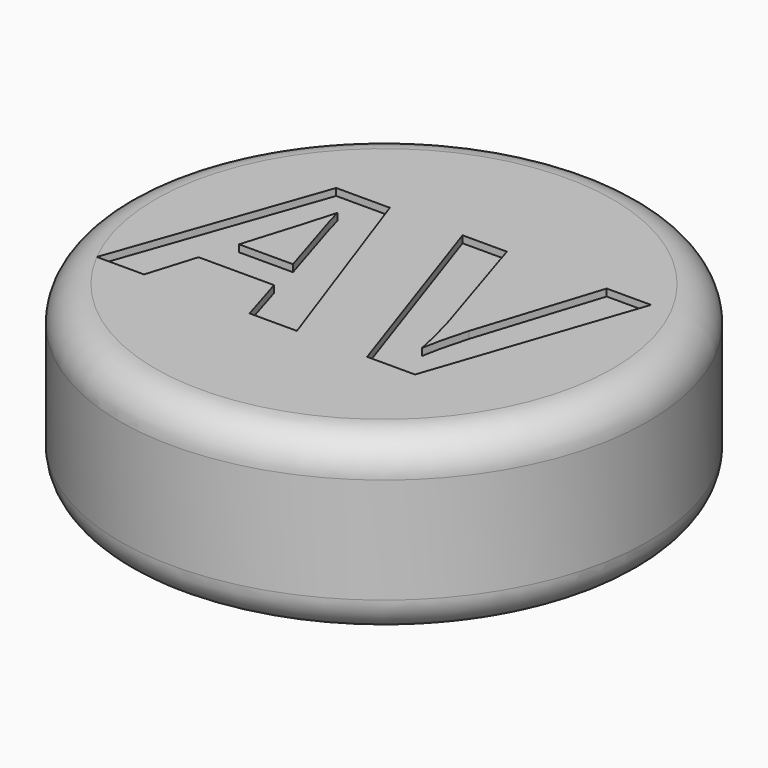
from build123d import *

# Parameters (mm, degrees)
F0_R         = 19.05
F1_DEPTH     = 12.7
F2_R         = 2.54
F3_TEXT_SIZE = 20.9190775202
F4_DEPTH     = 0.508


# Not quite as in the source:
# - Text() gives the source's letters only with a copy of the font that has no kerning and outlines rounded to 1/6400 em; it was checked with that copy


with BuildPart() as f1:
    # F0 (on Top) → F1 (new body)
    with BuildSketch(Plane.XY):
        Circle(F0_R)
    extrude(amount=F1_DEPTH)

    # F2
    f2_edges = [f1.edges().sort_by_distance(p)[0] for p in [
        (-19.05, 0, 0),
        (-19.05, 0, 12.7),
    ]]
    fillet(f2_edges, radius=F2_R)

    # F3 (on face) → F4 (cut)
    with BuildSketch(Plane.XY.offset(12.7)):
        with Locations((-14.692383352, -7.5308679073)):
            Text('AV', F3_TEXT_SIZE, font='Open Sans', font_style=FontStyle.BOLD, text_align=(TextAlign.LEFT, TextAlign.BOTTOM))
    extrude(amount=-F4_DEPTH, mode=Mode.SUBTRACT)


solid = f1.part
